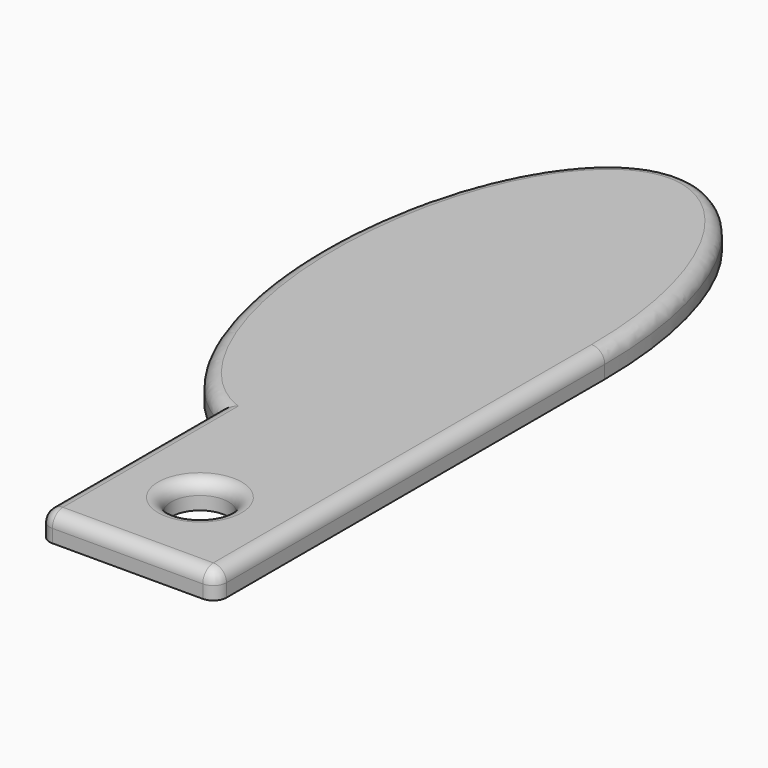
from build123d import *

# Parameters (mm, degrees)
F0_R        = 4.336036498
F1_DEPTH    = 4
F2_R        = 1.9999
F3_T1_DEPTH = 9
F3_T4_ANGLE = 90
F3_T6_ANGLE = 90


# Not quite as in the source:
# - a fillet or chamfer that OpenCascade refuses, or shapes differently, is made with other operations: its cross-section is extruded or revolved along the edge and cut away or added
# - a fillet or chamfer is up to 0.001 mm smaller than in the source, because OpenCascade refuses the exact size


with BuildPart() as f1:
    # F0 (on Top) → F1 (new body)
    with BuildSketch(Plane.XY):
        with BuildLine():
            add(Edge.make_bspline(
                [(-5.3302422166, -39.8106665894), (-2.7074100905, -41.0944335163), (0, -41.0944335163)],
                knots=[6.0325722383, 6.0325722383, 6.0325722383, 6.2831853072, 6.2831853072, 6.2831853072], degree=2, weights=[1, 0.9921594035, 1]))
            add(Edge.make_bspline(
                [(0, -41.0944335163), (21.4930921895, -41.0944335163), (21.4930921895, 0)],
                knots=[0, 0, 0, 1.5707963268, 1.5707963268, 1.5707963268], degree=2, weights=[1, 0.7071067812, 1]))
            add(Edge.make_bspline(
                [(21.4930921895, 0), (21.4930921895, 83.9221072153), (-13.1793327698, 32.4619744443), (-47.8517577291, -18.9981583267), (-5.3302422166, -39.8106665894)],
                knots=[1.5707963268, 1.5707963268, 1.5707963268, 3.8016842826, 3.8016842826, 6.0325722383, 6.0325722383, 6.0325722383], degree=2, weights=[1, 0.4397787878, 1, 0.4397787878, 1]))
        make_face()
        with BuildLine():
            add(Edge.make_bspline(
                [(0, -41.0944335163), (21.4930921895, -41.0944335163), (21.4930921895, 0)],
                knots=[0, 0, 0, 1.5707963268, 1.5707963268, 1.5707963268], degree=2, weights=[1, 0.7071067812, 1]))
            add(Edge.make_bspline(
                [(-5.3302422166, -39.8106665894), (-2.7074100905, -41.0944335163), (0, -41.0944335163)],
                knots=[6.0325722383, 6.0325722383, 6.0325722383, 6.2831853072, 6.2831853072, 6.2831853072], degree=2, weights=[1, 0.9921594035, 1]))
            Line((-5.3302422166, -39.8106665894), (-5.3302422166, -73.7636461854))
            Line((-5.3302422166, -73.7636461854), (21.4930921895, -73.7636461854))
            Line((21.4930921895, -73.7636461854), (21.4930921895, 0))
        make_face()
        with Locations((7.7548543923, -59.6359223127)):
            Circle(F0_R, mode=Mode.SUBTRACT)
    extrude(amount=-F1_DEPTH)

    # F2 (radius 2 in the source; OpenCascade refuses exactly that, so slightly less here)
    f2_edges = [f1.edges().sort_by_distance(p)[0] for p in [
        (-16.104761, 27.214024, 0),
        (-5.330242, -56.787156, 0),
        (8.081425, -73.763646, 0),
        (21.493092, -36.881823, 0),
        (3.418818, -59.635922, 0),
    ]]
    fillet(f2_edges, radius=F2_R)

    # F3: fillet of radius 2 on 2 edges, made by hand

    # F3_s2 → F3_t1 (cut)
    with BuildSketch(Plane.XY.offset(-9)):
        with BuildLine():
            ThreePointArc((21.4930921895, -71.7636461854), (20.9073057519, -73.1778597478), (19.4930921895, -73.7636461854))
            Line((19.4930921895, -73.7636461854), (21.4930921895, -73.7636461854))
            Line((21.4930921895, -73.7636461854), (21.4930921895, -71.7636461854))
        make_face()
        with BuildLine():
            ThreePointArc((-5.3302422166, -71.7636461854), (-4.744455779, -73.1778597478), (-3.3302422166, -73.7636461854))
            Line((-3.3302422166, -73.7636461854), (-5.3302422166, -73.7636461854))
            Line((-5.3302422166, -73.7636461854), (-5.3302422166, -71.7636461854))
        make_face()
    extrude(amount=F3_T1_DEPTH, mode=Mode.SUBTRACT)

    # F3_s3 → F3_t4 (revolve, cut)
    with BuildSketch(Plane.XZ.offset(71.7636461854)):
        with BuildLine():
            ThreePointArc((-3.3303422166, 0), (-4.7444850683, -0.5857571483), (-5.3302422166, -1.9999))
            Line((-5.3302422166, -1.9999), (-5.3302422166, 0))
            Line((-5.3302422166, 0), (-3.3303422166, 0))
        make_face()
    revolve(axis=Axis((-3.3302422166, -71.7636461854, 0), (0, 0, 1)), revolution_arc=F3_T4_ANGLE, mode=Mode.SUBTRACT)

    # F3_s5 → F3_t6 (revolve, cut)
    with BuildSketch(Plane.YZ.offset(19.4930921895)):
        with BuildLine():
            ThreePointArc((-71.7637461854, 0), (-73.1778890371, -0.5857571483), (-73.7636461854, -1.9999))
            Line((-73.7636461854, -1.9999), (-73.7636461854, 0))
            Line((-73.7636461854, 0), (-71.7637461854, 0))
        make_face()
    revolve(axis=Axis((19.4930921895, -71.7636461854, 0), (0, 0, 1)), revolution_arc=F3_T6_ANGLE, mode=Mode.SUBTRACT)


solid = f1.part
